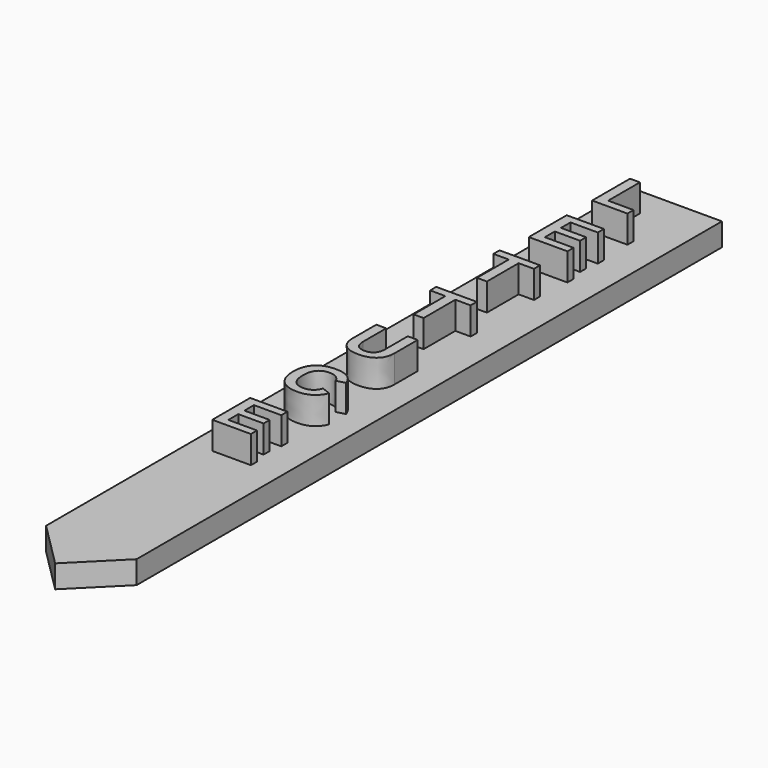
from build123d import *

# Parameters (mm, degrees)
F1_DEPTH     = 2.5
F2_TEXT_SIZE = 7.524023717
F3_DEPTH     = 3


# Not quite as in the source:
# - Text() gives the source's letters only with a copy of the font that has no kerning and outlines rounded to 1/6400 em; it was checked with that copy


with BuildPart() as f1:
    # F0 (on Top) → F1 (new body)
    with BuildSketch(Plane.XY):
        Polygon((-4.9497474683, 4.9497474683), (0, 0), (4.9497474683, 4.9497474683), (4.9497474683, 84.9497474683), (-4.9497474683, 84.9497474683), align=None)
    extrude(amount=F1_DEPTH)

    # F2 (on face) → F3 (join)
    with BuildSketch(Plane.XY.offset(2.5)):
        with Locations((-3.0119462958, 76.532450392)):
            Text('L', F2_TEXT_SIZE, font='Arimo', font_style=FontStyle.BOLD, text_align=(TextAlign.LEFT, TextAlign.BOTTOM))
        with Locations((-3.0119462958, 67.8798231175)):
            Text('E', F2_TEXT_SIZE, font='Arimo', font_style=FontStyle.BOLD, text_align=(TextAlign.LEFT, TextAlign.BOTTOM))
        with Locations((-3.0119462958, 59.2271958429)):
            Text('T', F2_TEXT_SIZE, font='Arimo', font_style=FontStyle.BOLD, text_align=(TextAlign.LEFT, TextAlign.BOTTOM))
        with Locations((-3.0119462958, 50.5745685683)):
            Text('T', F2_TEXT_SIZE, font='Arimo', font_style=FontStyle.BOLD, text_align=(TextAlign.LEFT, TextAlign.BOTTOM))
        with Locations((-3.0119462958, 41.9219412937)):
            Text('U', F2_TEXT_SIZE, font='Arimo', font_style=FontStyle.BOLD, text_align=(TextAlign.LEFT, TextAlign.BOTTOM))
        with Locations((-3.0119462958, 33.2693140191)):
            Text('C', F2_TEXT_SIZE, font='Arimo', font_style=FontStyle.BOLD, text_align=(TextAlign.LEFT, TextAlign.BOTTOM))
        with Locations((-3.0119462958, 24.6166867445)):
            Text('E', F2_TEXT_SIZE, font='Arimo', font_style=FontStyle.BOLD, text_align=(TextAlign.LEFT, TextAlign.BOTTOM))
    extrude(amount=F3_DEPTH)


solid = f1.part
